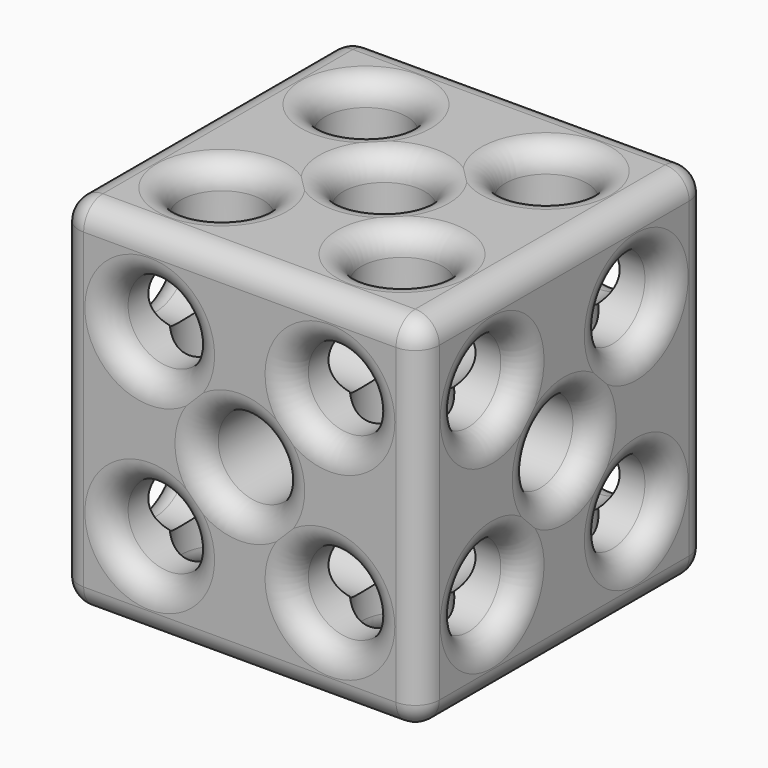
from build123d import *

# Parameters (mm, degrees)
F0_W         = 150
F0_H         = 150
F0_R         = 17
F1_DEPTH     = 150
F2_R         = 17
F3_DEPTH     = 150
F4_R         = 17
F5_DEPTH     = 150
F6_T1_DEPTH  = 130
F6_T3_DEPTH  = 130
F6_T5_DEPTH  = 130
F6_S9_W      = 10
F6_S9_H      = 10
F6_T10_DEPTH = 10
F6_S15_W     = 10
F6_S15_H     = 10
F6_T16_DEPTH = 10
F6_S21_W     = 10
F6_S21_H     = 10
F6_T22_DEPTH = 10
F6_S27_W     = 10
F6_S27_H     = 10
F6_T28_DEPTH = 10
F6_S33_W     = 10
F6_S33_H     = 10
F6_T34_DEPTH = 10
F6_S39_W     = 10
F6_S39_H     = 10
F6_T40_DEPTH = 10
F6_S45_W     = 10
F6_S45_H     = 10
F6_T46_DEPTH = 10
F6_S51_W     = 10
F6_S51_H     = 10
F6_T52_DEPTH = 10


# Not quite as in the source:
# - a fillet or chamfer that OpenCascade refuses, or shapes differently, is made with other operations: its cross-section is extruded or revolved along the edge and cut away or added


with BuildPart() as f1:
    # F0 (on Top) → F1 (new body)
    with BuildSketch(Plane.XY):
        Rectangle(F0_W, F0_H)
        with Locations((-37.5, -37.5)):
            Circle(F0_R, mode=Mode.SUBTRACT)
        with Locations((37.5, -37.5)):
            Circle(F0_R, mode=Mode.SUBTRACT)
        with Locations((-37.5, 37.5)):
            Circle(F0_R, mode=Mode.SUBTRACT)
        Circle(F0_R, mode=Mode.SUBTRACT)
        with Locations((37.5, 37.5)):
            Circle(F0_R, mode=Mode.SUBTRACT)
    extrude(amount=F1_DEPTH)

    # F2 (on face) → F3 (cut)
    with BuildSketch(Plane.XZ.offset(75)):
        with Locations((-37.5, 112.5)):
            Circle(F2_R)
        with Locations((-37.5, 37.5)):
            Circle(F2_R)
        with Locations((0, 75)):
            Circle(F2_R)
        with Locations((37.5, 37.5)):
            Circle(F2_R)
        with Locations((37.5, 112.5)):
            Circle(F2_R)
    extrude(amount=-F3_DEPTH, mode=Mode.SUBTRACT)

    # F4 (on face) → F5 (cut)
    with BuildSketch(Plane(origin=(-75, 0, 0), x_dir=(0, -1, 0), z_dir=(-1, 0, 0))):
        with Locations((-37.5, 37.5)):
            Circle(F4_R)
        with Locations((0, 75)):
            Circle(F4_R)
        with Locations((-37.5, 112.5)):
            Circle(F4_R)
        with Locations((37.5, 112.5)):
            Circle(F4_R)
        with Locations((37.5, 37.5)):
            Circle(F4_R)
    extrude(amount=-F5_DEPTH, mode=Mode.SUBTRACT)

    # F6: fillet of radius 10 on 42 edges, made by hand

    # F6_s2 → F6_t1 (cut)
    with BuildSketch(Plane.XY.offset(10)):
        with BuildLine():
            ThreePointArc((75, -65), (72.0710678119, -72.0710678119), (65, -75))
            Line((65, -75), (75, -75))
            Line((75, -75), (75, -65))
        make_face()
        with BuildLine():
            ThreePointArc((75, 65), (72.0710678119, 72.0710678119), (65, 75))
            Line((65, 75), (75, 75))
            Line((75, 75), (75, 65))
        make_face()
        with BuildLine():
            ThreePointArc((-65, -75), (-72.0710678119, -72.0710678119), (-75, -65))
            Line((-75, -65), (-75, -75))
            Line((-75, -75), (-65, -75))
        make_face()
        with BuildLine():
            ThreePointArc((-65, 75), (-72.0710678119, 72.0710678119), (-75, 65))
            Line((-75, 65), (-75, 75))
            Line((-75, 75), (-65, 75))
        make_face()
    extrude(amount=F6_T1_DEPTH, mode=Mode.SUBTRACT)

    # F6_s4 → F6_t3 (cut)
    with BuildSketch(Plane.XZ.offset(-65)):
        with BuildLine():
            ThreePointArc((75, 10), (72.0710678119, 2.9289321881), (65, 0))
            Line((65, 0), (75, 0))
            Line((75, 0), (75, 10))
        make_face()
        with BuildLine():
            ThreePointArc((75, 140), (72.0710678119, 147.0710678119), (65, 150))
            Line((65, 150), (75, 150))
            Line((75, 150), (75, 140))
        make_face()
        with BuildLine():
            ThreePointArc((-65, 150), (-72.0710678119, 147.0710678119), (-75, 140))
            Line((-75, 140), (-75, 150))
            Line((-75, 150), (-65, 150))
        make_face()
        with BuildLine():
            ThreePointArc((-65, 0), (-72.0710678119, 2.9289321881), (-75, 10))
            Line((-75, 10), (-75, 0))
            Line((-75, 0), (-65, 0))
        make_face()
    extrude(amount=F6_T3_DEPTH, mode=Mode.SUBTRACT)

    # F6_s6 → F6_t5 (cut)
    with BuildSketch(Plane.YZ.offset(-65)):
        with BuildLine():
            ThreePointArc((65, 150), (72.0710678119, 147.0710678119), (75, 140))
            Line((75, 140), (75, 150))
            Line((75, 150), (65, 150))
        make_face()
        with BuildLine():
            ThreePointArc((-75, 140), (-72.0710678119, 147.0710678119), (-65, 150))
            Line((-65, 150), (-75, 150))
            Line((-75, 150), (-75, 140))
        make_face()
        with BuildLine():
            ThreePointArc((-75, 10), (-72.0710678119, 2.9289321881), (-65, 0))
            Line((-65, 0), (-75, 0))
            Line((-75, 0), (-75, 10))
        make_face()
        with BuildLine():
            ThreePointArc((65, 0), (72.0710678119, 2.9289321881), (75, 10))
            Line((75, 10), (75, 0))
            Line((75, 0), (65, 0))
        make_face()
    extrude(amount=F6_T5_DEPTH, mode=Mode.SUBTRACT)


with BuildPart() as f6_tool8:
    # F6_s9 → F6_t10 (new body)
    with BuildSketch(Plane.YZ.offset(65)):
        with Locations((-70, 5)):
            Rectangle(F6_S9_W, F6_S9_H)
    extrude(amount=F6_T10_DEPTH)

    # F6_s11 → F6_t12 (revolve, cut)
    with BuildSketch(Plane(origin=(65, -65, 10), x_dir=(0, 0.7071067812, 0.7071067812), z_dir=(0, 0.7071067812, -0.7071067812))):
        with BuildLine():
            ThreePointArc((0, -10), (10, 0), (0, 10))
            Line((0, 10), (0, -10))
        make_face()
    revolve(axis=Axis((65, -65, 10), (1, 0, 0)), mode=Mode.SUBTRACT)


with BuildPart() as f1_1:
    add(f1.part)

    # F6_t7: cut F6_tool8
    add(f6_tool8.part, mode=Mode.SUBTRACT)


with BuildPart() as f6_tool14:
    # F6_s15 → F6_t16 (new body)
    with BuildSketch(Plane.YZ.offset(65)):
        with Locations((-70, 145)):
            Rectangle(F6_S15_W, F6_S15_H)
    extrude(amount=F6_T16_DEPTH)

    # F6_s17 → F6_t18 (revolve, cut)
    with BuildSketch(Plane(origin=(65, -65, 140), x_dir=(0, 0.7071067812, -0.7071067812), z_dir=(0, -0.7071067812, -0.7071067812))):
        with BuildLine():
            ThreePointArc((0, -10), (10, 0), (0, 10))
            Line((0, 10), (0, -10))
        make_face()
    revolve(axis=Axis((65, -65, 140), (1, 0, 0)), mode=Mode.SUBTRACT)


with BuildPart() as f1_2:
    add(f1_1.part)

    # F6_t13: cut F6_tool14
    add(f6_tool14.part, mode=Mode.SUBTRACT)


with BuildPart() as f6_tool20:
    # F6_s21 → F6_t22 (new body)
    with BuildSketch(Plane.YZ.offset(65)):
        with Locations((70, 5)):
            Rectangle(F6_S21_W, F6_S21_H)
    extrude(amount=F6_T22_DEPTH)

    # F6_s23 → F6_t24 (revolve, cut)
    with BuildSketch(Plane(origin=(65, 65, 10), x_dir=(0, -0.7071067812, 0.7071067812), z_dir=(0, 0.7071067812, 0.7071067812))):
        with BuildLine():
            ThreePointArc((0, -10), (10, 0), (0, 10))
            Line((0, 10), (0, -10))
        make_face()
    revolve(axis=Axis((65, 65, 10), (1, 0, 0)), mode=Mode.SUBTRACT)


with BuildPart() as f1_3:
    add(f1_2.part)

    # F6_t19: cut F6_tool20
    add(f6_tool20.part, mode=Mode.SUBTRACT)


with BuildPart() as f6_tool26:
    # F6_s27 → F6_t28 (new body)
    with BuildSketch(Plane.YZ.offset(65)):
        with Locations((70, 145)):
            Rectangle(F6_S27_W, F6_S27_H)
    extrude(amount=F6_T28_DEPTH)

    # F6_s29 → F6_t30 (revolve, cut)
    with BuildSketch(Plane(origin=(65, 65, 140), x_dir=(0, -0.7071067812, -0.7071067812), z_dir=(0, -0.7071067812, 0.7071067812))):
        with BuildLine():
            ThreePointArc((0, -10), (10, 0), (0, 10))
            Line((0, 10), (0, -10))
        make_face()
    revolve(axis=Axis((65, 65, 140), (1, 0, 0)), mode=Mode.SUBTRACT)


with BuildPart() as f1_4:
    add(f1_3.part)

    # F6_t25: cut F6_tool26
    add(f6_tool26.part, mode=Mode.SUBTRACT)


with BuildPart() as f6_tool32:
    # F6_s33 → F6_t34 (new body)
    with BuildSketch(Plane.YZ.offset(-65)):
        with Locations((70, 145)):
            Rectangle(F6_S33_W, F6_S33_H)
    extrude(amount=-F6_T34_DEPTH)

    # F6_s35 → F6_t36 (revolve, cut)
    with BuildSketch(Plane(origin=(-65, 65, 140), x_dir=(0, -0.7071067812, -0.7071067812), z_dir=(0, 0.7071067812, -0.7071067812))):
        with BuildLine():
            ThreePointArc((0, -10), (10, 0), (0, 10))
            Line((0, 10), (0, -10))
        make_face()
    revolve(axis=Axis((-65, 65, 140), (-1, 0, 0)), mode=Mode.SUBTRACT)


with BuildPart() as f1_5:
    add(f1_4.part)

    # F6_t31: cut F6_tool32
    add(f6_tool32.part, mode=Mode.SUBTRACT)


with BuildPart() as f6_tool38:
    # F6_s39 → F6_t40 (new body)
    with BuildSketch(Plane.XZ.offset(65)):
        with Locations((-70, 145)):
            Rectangle(F6_S39_W, F6_S39_H)
    extrude(amount=F6_T40_DEPTH)

    # F6_s41 → F6_t42 (revolve, cut)
    with BuildSketch(Plane(origin=(-65, -65, 140), x_dir=(0.7071067812, 0, -0.7071067812), z_dir=(-0.7071067812, 0, -0.7071067812))):
        with BuildLine():
            ThreePointArc((0, -10), (10, 0), (0, 10))
            Line((0, 10), (0, -10))
        make_face()
    revolve(axis=Axis((-65, -65, 140), (0, -1, 0)), mode=Mode.SUBTRACT)


with BuildPart() as f1_6:
    add(f1_5.part)

    # F6_t37: cut F6_tool38
    add(f6_tool38.part, mode=Mode.SUBTRACT)


with BuildPart() as f6_tool44:
    # F6_s45 → F6_t46 (new body)
    with BuildSketch(Plane.XZ.offset(65)):
        with Locations((-70, 5)):
            Rectangle(F6_S45_W, F6_S45_H)
    extrude(amount=F6_T46_DEPTH)

    # F6_s47 → F6_t48 (revolve, cut)
    with BuildSketch(Plane(origin=(-65, -65, 10), x_dir=(0.7071067812, 0, 0.7071067812), z_dir=(0.7071067812, 0, -0.7071067812))):
        with BuildLine():
            ThreePointArc((0, -10), (10, 0), (0, 10))
            Line((0, 10), (0, -10))
        make_face()
    revolve(axis=Axis((-65, -65, 10), (0, -1, 0)), mode=Mode.SUBTRACT)


with BuildPart() as f1_7:
    add(f1_6.part)

    # F6_t43: cut F6_tool44
    add(f6_tool44.part, mode=Mode.SUBTRACT)


with BuildPart() as f6_tool50:
    # F6_s51 → F6_t52 (new body)
    with BuildSketch(Plane.XY.offset(10)):
        with Locations((-70, 70)):
            Rectangle(F6_S51_W, F6_S51_H)
    extrude(amount=-F6_T52_DEPTH)

    # F6_s53 → F6_t54 (revolve, cut)
    with BuildSketch(Plane(origin=(-65, 65, 10), x_dir=(0.7071067812, -0.7071067812, 0), z_dir=(0.7071067812, 0.7071067812, 0))):
        with BuildLine():
            ThreePointArc((0, -10), (10, 0), (0, 10))
            Line((0, 10), (0, -10))
        make_face()
    revolve(axis=Axis((-65, 65, 10), (0, 0, -1)), mode=Mode.SUBTRACT)


with BuildPart() as f1_8:
    add(f1_7.part)

    # F6_t49: cut F6_tool50
    add(f6_tool50.part, mode=Mode.SUBTRACT)

    # F6_s55 → F6_t56 (revolve, cut)
    with BuildSketch(Plane.XY.offset(112.5)):
        with BuildLine():
            ThreePointArc((75, -64.5), (72.0710678119, -57.4289321881), (65, -54.5))
            Line((65, -54.5), (75, -54.5))
            Line((75, -54.5), (75, -64.5))
        make_face()
    revolve(axis=Axis((75, -37.5, 112.5), (-1, 0, 0)), mode=Mode.SUBTRACT)

    # F6_s57 → F6_t58 (revolve, cut)
    with BuildSketch(Plane.XY.offset(112.5)):
        with BuildLine():
            ThreePointArc((75, 10.5), (72.0710678119, 17.5710678119), (65, 20.5))
            Line((65, 20.5), (75, 20.5))
            Line((75, 20.5), (75, 10.5))
        make_face()
    revolve(axis=Axis((75, 37.5, 112.5), (-1, 0, 0)), mode=Mode.SUBTRACT)

    # F6_s59 → F6_t60 (revolve, cut)
    with BuildSketch(Plane.XY.offset(37.5)):
        with BuildLine():
            ThreePointArc((75, -64.5), (72.0710678119, -57.4289321881), (65, -54.5))
            Line((65, -54.5), (75, -54.5))
            Line((75, -54.5), (75, -64.5))
        make_face()
    revolve(axis=Axis((75, -37.5, 37.5), (-1, 0, 0)), mode=Mode.SUBTRACT)

    # F6_s61 → F6_t62 (revolve, cut)
    with BuildSketch(Plane.XY.offset(75)):
        with BuildLine():
            ThreePointArc((75, -27), (72.0710678119, -19.9289321881), (65, -17))
            Line((65, -17), (75, -17))
            Line((75, -17), (75, -27))
        make_face()
    revolve(axis=Axis((75, 0, 75), (-1, 0, 0)), mode=Mode.SUBTRACT)

    # F6_s63 → F6_t64 (revolve, cut)
    with BuildSketch(Plane.XY.offset(37.5)):
        with BuildLine():
            ThreePointArc((75, 10.5), (72.0710678119, 17.5710678119), (65, 20.5))
            Line((65, 20.5), (75, 20.5))
            Line((75, 20.5), (75, 10.5))
        make_face()
    revolve(axis=Axis((75, 37.5, 37.5), (-1, 0, 0)), mode=Mode.SUBTRACT)

    # F6_s65 → F6_t66 (revolve, cut)
    with BuildSketch(Plane.XZ.offset(37.5)):
        with BuildLine():
            ThreePointArc((-10.5, 150), (-17.5710678119, 147.0710678119), (-20.5, 140))
            Line((-20.5, 140), (-20.5, 150))
            Line((-20.5, 150), (-10.5, 150))
        make_face()
    revolve(axis=Axis((-37.5, -37.5, 150), (0, 0, 1)), mode=Mode.SUBTRACT)

    # F6_s67 → F6_t68 (revolve, cut)
    with BuildSketch(Plane.XZ.offset(37.5)):
        with BuildLine():
            ThreePointArc((64.5, 150), (57.4289321881, 147.0710678119), (54.5, 140))
            Line((54.5, 140), (54.5, 150))
            Line((54.5, 150), (64.5, 150))
        make_face()
    revolve(axis=Axis((37.5, -37.5, 150), (0, 0, 1)), mode=Mode.SUBTRACT)

    # F6_s69 → F6_t70 (revolve, cut)
    with BuildSketch(Plane.XZ.offset(-37.5)):
        with BuildLine():
            ThreePointArc((-10.5, 150), (-17.5710678119, 147.0710678119), (-20.5, 140))
            Line((-20.5, 140), (-20.5, 150))
            Line((-20.5, 150), (-10.5, 150))
        make_face()
    revolve(axis=Axis((-37.5, 37.5, 150), (0, 0, 1)), mode=Mode.SUBTRACT)

    # F6_s71 → F6_t72 (revolve, cut)
    with BuildSketch(Plane.XZ):
        with BuildLine():
            ThreePointArc((27, 150), (19.9289321881, 147.0710678119), (17, 140))
            Line((17, 140), (17, 150))
            Line((17, 150), (27, 150))
        make_face()
    revolve(axis=Axis((0, 0, 150), (0, 0, 1)), mode=Mode.SUBTRACT)

    # F6_s73 → F6_t74 (revolve, cut)
    with BuildSketch(Plane.XZ.offset(-37.5)):
        with BuildLine():
            ThreePointArc((64.5, 150), (57.4289321881, 147.0710678119), (54.5, 140))
            Line((54.5, 140), (54.5, 150))
            Line((54.5, 150), (64.5, 150))
        make_face()
    revolve(axis=Axis((37.5, 37.5, 150), (0, 0, 1)), mode=Mode.SUBTRACT)

    # F6_s75 → F6_t76 (revolve, cut)
    with BuildSketch(Plane.XY.offset(112.5)):
        with BuildLine():
            ThreePointArc((-10.5, -75), (-17.5710678119, -72.0710678119), (-20.5, -65))
            Line((-20.5, -65), (-20.5, -75))
            Line((-20.5, -75), (-10.5, -75))
        make_face()
    revolve(axis=Axis((-37.5, -75, 112.5), (0, -1, 0)), mode=Mode.SUBTRACT)

    # F6_s77 → F6_t78 (revolve, cut)
    with BuildSketch(Plane.XY.offset(112.5)):
        with BuildLine():
            ThreePointArc((64.5, -75), (57.4289321881, -72.0710678119), (54.5, -65))
            Line((54.5, -65), (54.5, -75))
            Line((54.5, -75), (64.5, -75))
        make_face()
    revolve(axis=Axis((37.5, -75, 112.5), (0, -1, 0)), mode=Mode.SUBTRACT)

    # F6_s79 → F6_t80 (revolve, cut)
    with BuildSketch(Plane.XY.offset(37.5)):
        with BuildLine():
            ThreePointArc((-10.5, -75), (-17.5710678119, -72.0710678119), (-20.5, -65))
            Line((-20.5, -65), (-20.5, -75))
            Line((-20.5, -75), (-10.5, -75))
        make_face()
    revolve(axis=Axis((-37.5, -75, 37.5), (0, -1, 0)), mode=Mode.SUBTRACT)

    # F6_s81 → F6_t82 (revolve, cut)
    with BuildSketch(Plane.XY.offset(75)):
        with BuildLine():
            ThreePointArc((27, -75), (19.9289321881, -72.0710678119), (17, -65))
            Line((17, -65), (17, -75))
            Line((17, -75), (27, -75))
        make_face()
    revolve(axis=Axis((0, -75, 75), (0, -1, 0)), mode=Mode.SUBTRACT)

    # F6_s83 → F6_t84 (revolve, cut)
    with BuildSketch(Plane.XY.offset(37.5)):
        with BuildLine():
            ThreePointArc((64.5, -75), (57.4289321881, -72.0710678119), (54.5, -65))
            Line((54.5, -65), (54.5, -75))
            Line((54.5, -75), (64.5, -75))
        make_face()
    revolve(axis=Axis((37.5, -75, 37.5), (0, -1, 0)), mode=Mode.SUBTRACT)

    # F6_s85 → F6_t86 (revolve, cut)
    with BuildSketch(Plane.XZ.offset(37.5)):
        with BuildLine():
            ThreePointArc((-10.5, 0), (-17.5710678119, 2.9289321881), (-20.5, 10))
            Line((-20.5, 10), (-20.5, 0))
            Line((-20.5, 0), (-10.5, 0))
        make_face()
    revolve(axis=Axis((-37.5, -37.5, 0), (0, 0, 1)), mode=Mode.SUBTRACT)

    # F6_s87 → F6_t88 (revolve, cut)
    with BuildSketch(Plane.XZ.offset(37.5)):
        with BuildLine():
            ThreePointArc((64.5, 0), (57.4289321881, 2.9289321881), (54.5, 10))
            Line((54.5, 10), (54.5, 0))
            Line((54.5, 0), (64.5, 0))
        make_face()
    revolve(axis=Axis((37.5, -37.5, 0), (0, 0, 1)), mode=Mode.SUBTRACT)

    # F6_s89 → F6_t90 (revolve, cut)
    with BuildSketch(Plane.XZ.offset(-37.5)):
        with BuildLine():
            ThreePointArc((-10.5, 0), (-17.5710678119, 2.9289321881), (-20.5, 10))
            Line((-20.5, 10), (-20.5, 0))
            Line((-20.5, 0), (-10.5, 0))
        make_face()
    revolve(axis=Axis((-37.5, 37.5, 0), (0, 0, 1)), mode=Mode.SUBTRACT)

    # F6_s91 → F6_t92 (revolve, cut)
    with BuildSketch(Plane.XZ):
        with BuildLine():
            ThreePointArc((27, 0), (19.9289321881, 2.9289321881), (17, 10))
            Line((17, 10), (17, 0))
            Line((17, 0), (27, 0))
        make_face()
    revolve(axis=Axis((0, 0, 0), (0, 0, 1)), mode=Mode.SUBTRACT)

    # F6_s93 → F6_t94 (revolve, cut)
    with BuildSketch(Plane.XZ.offset(-37.5)):
        with BuildLine():
            ThreePointArc((64.5, 0), (57.4289321881, 2.9289321881), (54.5, 10))
            Line((54.5, 10), (54.5, 0))
            Line((54.5, 0), (64.5, 0))
        make_face()
    revolve(axis=Axis((37.5, 37.5, 0), (0, 0, 1)), mode=Mode.SUBTRACT)

    # F6_s95 → F6_t96 (revolve, cut)
    with BuildSketch(Plane.XY.offset(112.5)):
        with BuildLine():
            ThreePointArc((64.5, 75), (57.4289321881, 72.0710678119), (54.5, 65))
            Line((54.5, 65), (54.5, 75))
            Line((54.5, 75), (64.5, 75))
        make_face()
    revolve(axis=Axis((37.5, 75, 112.5), (0, -1, 0)), mode=Mode.SUBTRACT)

    # F6_s97 → F6_t98 (revolve, cut)
    with BuildSketch(Plane.XY.offset(112.5)):
        with BuildLine():
            ThreePointArc((-10.5, 75), (-17.5710678119, 72.0710678119), (-20.5, 65))
            Line((-20.5, 65), (-20.5, 75))
            Line((-20.5, 75), (-10.5, 75))
        make_face()
    revolve(axis=Axis((-37.5, 75, 112.5), (0, -1, 0)), mode=Mode.SUBTRACT)

    # F6_s99 → F6_t100 (revolve, cut)
    with BuildSketch(Plane.XY.offset(37.5)):
        with BuildLine():
            ThreePointArc((64.5, 75), (57.4289321881, 72.0710678119), (54.5, 65))
            Line((54.5, 65), (54.5, 75))
            Line((54.5, 75), (64.5, 75))
        make_face()
    revolve(axis=Axis((37.5, 75, 37.5), (0, -1, 0)), mode=Mode.SUBTRACT)

    # F6_s101 → F6_t102 (revolve, cut)
    with BuildSketch(Plane.XY.offset(75)):
        with BuildLine():
            ThreePointArc((27, 75), (19.9289321881, 72.0710678119), (17, 65))
            Line((17, 65), (17, 75))
            Line((17, 75), (27, 75))
        make_face()
    revolve(axis=Axis((0, 75, 75), (0, -1, 0)), mode=Mode.SUBTRACT)

    # F6_s103 → F6_t104 (revolve, cut)
    with BuildSketch(Plane.XY.offset(37.5)):
        with BuildLine():
            ThreePointArc((-10.5, 75), (-17.5710678119, 72.0710678119), (-20.5, 65))
            Line((-20.5, 65), (-20.5, 75))
            Line((-20.5, 75), (-10.5, 75))
        make_face()
    revolve(axis=Axis((-37.5, 75, 37.5), (0, -1, 0)), mode=Mode.SUBTRACT)

    # F6_s105 → F6_t106 (revolve, cut)
    with BuildSketch(Plane.XY.offset(112.5)):
        with BuildLine():
            ThreePointArc((-75, 10.5), (-72.0710678119, 17.5710678119), (-65, 20.5))
            Line((-65, 20.5), (-75, 20.5))
            Line((-75, 20.5), (-75, 10.5))
        make_face()
    revolve(axis=Axis((-75, 37.5, 112.5), (-1, 0, 0)), mode=Mode.SUBTRACT)

    # F6_s107 → F6_t108 (revolve, cut)
    with BuildSketch(Plane.XY.offset(112.5)):
        with BuildLine():
            ThreePointArc((-75, -64.5), (-72.0710678119, -57.4289321881), (-65, -54.5))
            Line((-65, -54.5), (-75, -54.5))
            Line((-75, -54.5), (-75, -64.5))
        make_face()
    revolve(axis=Axis((-75, -37.5, 112.5), (-1, 0, 0)), mode=Mode.SUBTRACT)

    # F6_s109 → F6_t110 (revolve, cut)
    with BuildSketch(Plane.XY.offset(37.5)):
        with BuildLine():
            ThreePointArc((-75, 10.5), (-72.0710678119, 17.5710678119), (-65, 20.5))
            Line((-65, 20.5), (-75, 20.5))
            Line((-75, 20.5), (-75, 10.5))
        make_face()
    revolve(axis=Axis((-75, 37.5, 37.5), (-1, 0, 0)), mode=Mode.SUBTRACT)

    # F6_s111 → F6_t112 (revolve, cut)
    with BuildSketch(Plane.XY.offset(75)):
        with BuildLine():
            ThreePointArc((-75, -27), (-72.0710678119, -19.9289321881), (-65, -17))
            Line((-65, -17), (-75, -17))
            Line((-75, -17), (-75, -27))
        make_face()
    revolve(axis=Axis((-75, 0, 75), (-1, 0, 0)), mode=Mode.SUBTRACT)

    # F6_s113 → F6_t114 (revolve, cut)
    with BuildSketch(Plane.XY.offset(37.5)):
        with BuildLine():
            ThreePointArc((-75, -64.5), (-72.0710678119, -57.4289321881), (-65, -54.5))
            Line((-65, -54.5), (-75, -54.5))
            Line((-75, -54.5), (-75, -64.5))
        make_face()
    revolve(axis=Axis((-75, -37.5, 37.5), (-1, 0, 0)), mode=Mode.SUBTRACT)


solid = f1_8.part
